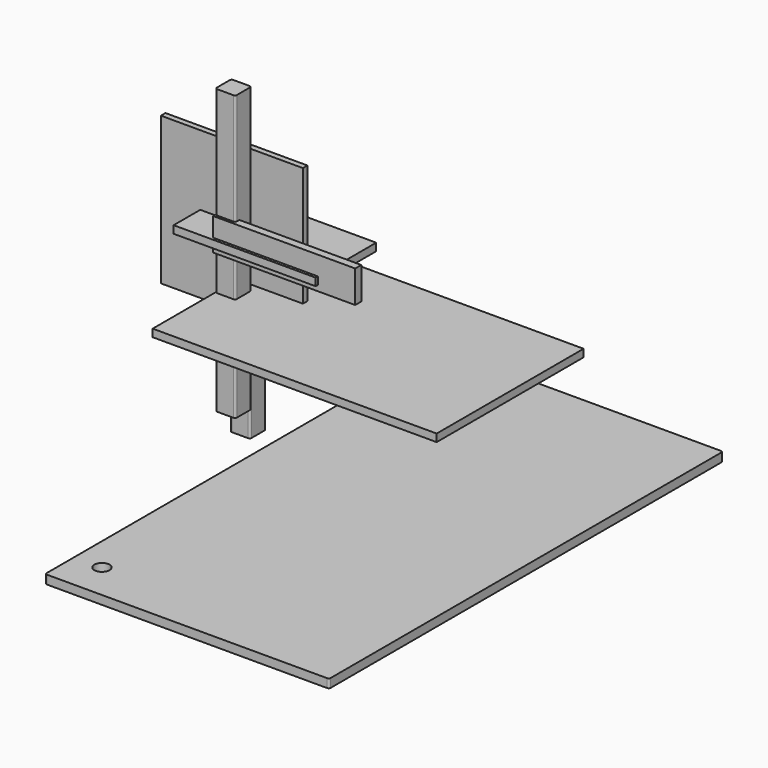
from build123d import *

# Parameters (mm, degrees)
F1_DEPTH        = 750
F3_DEPTH        = 53
F5_DEPTH        = 53
F6_R            = 5
F6_2_R          = 5
F6_3_R          = 5
F7_R            = 5
F9_W            = 375
F9_H            = 390
F10_DEPTH       = 15
F11_W           = 375
F11_H           = 200
F12_DEPTH       = 20
F13_W           = 485
F13_H           = 20
F14_DEPTH       = 750
F16_D           = 40
F16_DEPTH       = 40
F16_CBORE_D     = 40
F16_CBORE_DEPTH = 5
F16_TIP         = 12.0172123806
F17_W           = 20
F17_H           = 85
F18_DEPTH       = 375


# Not quite as in the source:
# - two fillets or chamfers of one size are made in one step


with BuildPart() as f1:
    # F0 (on Right) → F1 (new body)
    with BuildSketch(Plane.YZ):
        Polygon((649.3892060593, -536.194252491), (-650.6107939407, -536.194252491), (-650.6107939407, -559.194252491), (-635.6107939407, -559.194252491), (-435.6107939407, -559.194252491), (-420.6107939407, -559.194252491), (-417.3657000065, -559.194252491), (-399.3657000065, -559.194252491), (549.3892060593, -559.194252491), (569.3892060593, -559.194252491), (649.3892060593, -559.194252491), align=None)
    extrude(amount=F1_DEPTH)

    # F6
    f6_edges = [f1.edges().sort_by_distance(p)[0] for p in [
        (750, -650.610794, -547.694252),
        (750, 649.389206, -547.694252),
        (0, 649.389206, -547.694252),
        (0, -650.610794, -547.694252),
    ]]
    fillet(f6_edges, radius=F6_R)

    # F16
    with Locations(Plane.XY.offset(-536.194252491)):
        with Locations((73.1676146388, -554.3999671936)):
            CounterBoreHole(F16_D / 2, F16_CBORE_D / 2, F16_CBORE_DEPTH, depth=F16_DEPTH)
            with Locations((0, 0, -(F16_DEPTH + F16_TIP / 2))):  # 118° drill point
                Cone(0, F16_D / 2, F16_TIP, mode=Mode.SUBTRACT)


with BuildPart() as f3:
    # F2 (on Right) → F3 (new body)
    with BuildSketch(Plane.YZ):
        Polygon((-35.8609634377, 364.1842640936), (-88.8609634377, 364.1842640936), (-88.8609634377, 341.5341340936), (-88.8609634377, 142.1397668123), (-88.8609634377, 122.1397668123), (-88.8609634377, 4.1842640936), (-88.8609634377, -10.8157359064), (-88.8609634377, -385.8157359064), (-35.8609634377, -385.8157359064), align=None)
    extrude(amount=F3_DEPTH)

    # F6#2
    f6_2_edges = [f3.edges().sort_by_distance(p)[0] for p in [
        (53, -88.860963, -10.815736),
        (53, -35.860963, -10.815736),
        (0, -35.860963, -10.815736),
    ]]
    fillet(f6_2_edges, radius=F6_2_R)

    # F7
    f7_edges = [f3.edges().sort_by_distance(p)[0] for p in [
        (0, -88.860963, -10.815736),
    ]]
    fillet(f7_edges, radius=F7_R)


with BuildPart() as f5:
    # F4 (on Right) → F5 (new body)
    with BuildSketch(Plane.YZ):
        Polygon((12.5836707864, -115.9304558238), (-40.4163292136, -115.9304558238), (-40.4163292136, -138.5805858238), (-40.4163292136, -269.4304558238), (-40.4163292136, -284.4304558238), (-40.4163292136, -452.9304558238), (12.5836707864, -452.9304558238), align=None)
    extrude(amount=F5_DEPTH)

    # F6#3
    f6_3_edges = [f5.edges().sort_by_distance(p)[0] for p in [
        (0, 12.583671, -284.430456),
        (53, 12.583671, -284.430456),
        (53, -40.416329, -284.430456),
        (0, -40.416329, -284.430456),
    ]]
    fillet(f6_3_edges, radius=F6_3_R)


with BuildPart() as f10:
    # F9 (on Front) → F10 (new body)
    with BuildSketch(Plane.XZ):
        with Locations((-15.1590108871, 10.105997324)):
            Rectangle(F9_W, F9_H)
    extrude(amount=F10_DEPTH)


with BuildPart() as f12:
    # F11 (on Top) → F12 (new body)
    with BuildSketch(Plane.XY):
        with Locations((88.7996369725, -2.9512345791)):
            Rectangle(F11_W, F11_H)
    extrude(amount=F12_DEPTH)


with BuildPart() as f14:
    # F13 (on Right) → F14 (new body)
    with BuildSketch(Plane.YZ):
        with Locations((-53.0060548335, -120.13693689)):
            Rectangle(F13_W, F13_H)
    extrude(amount=F14_DEPTH)


with BuildPart() as f18:
    # F17 (on Right) → F18 (new body)
    with BuildSketch(Plane.YZ):
        with Locations((-85.6926859457, 27.9485643841)):
            Rectangle(F17_W, F17_H)
    extrude(amount=F18_DEPTH)


solid = Compound([f1.part, f3.part, f5.part, f10.part, f12.part, f14.part, f18.part])
